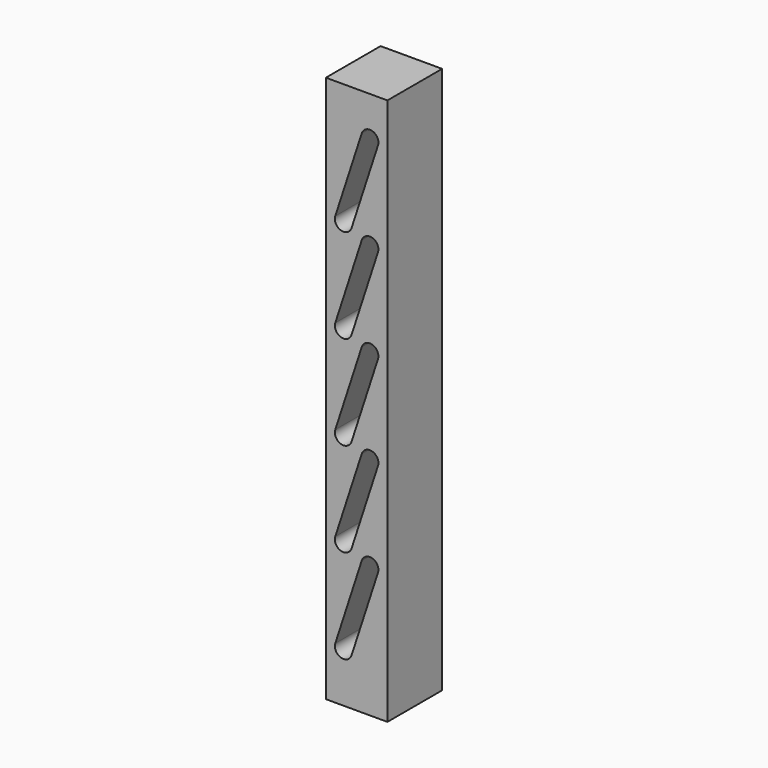
from build123d import *

# Parameters (mm, degrees)
F0_W     = 22.86
F0_H     = 203.2
F1_DEPTH = 25.4


# Not quite as in the source:
# - ends of sketch curves that miss each other by under 0.0002 mm in the source are joined


with BuildPart() as f1:
    # F0 (on Front) → F1 (new body)
    with BuildSketch(Plane.XZ):
        with Locations((-0.3399215189, 11.8189063548)):
            Rectangle(F0_W, F0_H)
        with BuildLine():
            Line((7.5848784811, -7.2097627448), (-2.2264276225, -37.4049924117))
            ThreePointArc((-2.2264276225, -37.4049924117), (-6.2271781929, -39.4434341876), (-8.2656199687, -35.4426836172))
            Line((-8.2656199687, -35.4426836172), (1.5459240038, -5.2467218859))
            ThreePointArc((1.5459240926, -5.2467219148), (5.5470406879, -3.2083990956), (7.5848784811, -7.2097627448))
        make_face(mode=Mode.SUBTRACT)
        with BuildLine():
            Line((7.5848784811, -42.1355889051), (-2.2258696668, -72.3299669673))
            ThreePointArc((-2.2258696668, -72.3299669673), (-6.2266030631, -74.3684424494), (-8.2650785452, -70.367709053))
            Line((-8.2650785452, -70.367709053), (1.5462110262, -40.1716646606))
            ThreePointArc((1.5462110262, -40.1716646606), (5.5477780101, -38.1334601546), (7.5848784811, -42.1355889051))
        make_face(mode=Mode.SUBTRACT)
        with BuildLine():
            Line((7.5848784811, 27.7160793915), (-2.2264110515, -2.4799669119))
            ThreePointArc((-2.2264110515, -2.4799669119), (-6.2271444076, -4.5184424731), (-8.2656199687, -0.517709117))
            Line((-8.2656199687, -0.517709117), (1.5456690059, 29.6783354693))
            ThreePointArc((1.5456690059, 29.6783354693), (5.5464015034, 31.7168113094), (7.5848784811, 27.7160793915))
        make_face(mode=Mode.SUBTRACT)
        with BuildLine():
            Line((7.5848784811, 97.5660773977), (-2.2264110903, 67.3700330053))
            ThreePointArc((-2.2264110903, 67.3700330053), (-6.2271444866, 65.3315575232), (-8.2656199687, 69.3322909196))
            Line((-8.2656199687, 69.3322909196), (1.5456696027, 99.528335312))
            ThreePointArc((1.5456696027, 99.528335312), (5.546402999, 101.5668107941), (7.5848784811, 97.5660773977))
        make_face(mode=Mode.SUBTRACT)
        with BuildLine():
            Line((7.5848784811, 62.6383122648), (-2.2255126404, 32.4450330169))
            ThreePointArc((-2.2255126404, 32.4450330169), (-6.2262460368, 30.4065575348), (-8.2647215189, 34.4072909311))
            Line((-8.2647215189, 34.4072909311), (1.5465680525, 64.6033353235))
            ThreePointArc((1.5465680525, 64.6033353235), (5.5486851845, 66.6413608527), (7.5848784811, 62.6383122648))
        make_face(mode=Mode.SUBTRACT)
    extrude(amount=F1_DEPTH)


solid = f1.part
